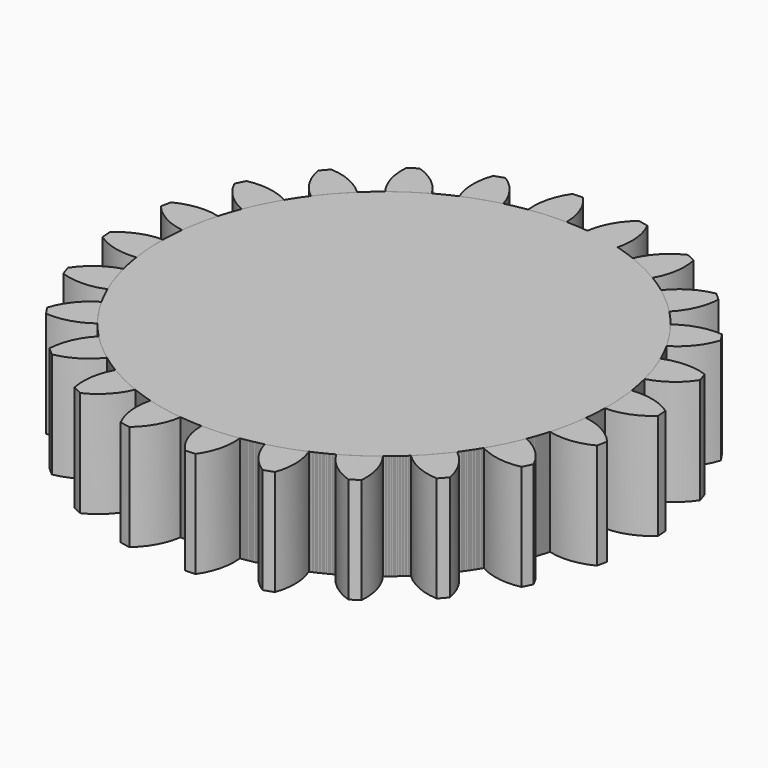
from build123d import *

# Parameters (mm, degrees)
F2_DEPTH = 1
F3_COUNT = 24
F3_ANGLE = 345


with BuildPart() as f2:
    # F1 (on Top) → F2 (new body)
    with BuildSketch(Plane.XY):
        with BuildLine():
            ThreePointArc((-0.3105516631, 2.0924649903), (-1.3816504371, -1.60184086), (2.1153846154, 0))
            ThreePointArc((2.1153846154, 0), (1.5080469337, 1.4834576222), (0.0347733631, 2.1150987883))
            ThreePointArc((0.0347733631, 2.1150987883), (-0.1383527734, 2.1108554145), (-0.3105516631, 2.0924649903))
        make_face()
        with BuildLine():
            ThreePointArc((-0.3105516631, 2.0924649903), (-0.1383527734, 2.1108554145), (0.0347733631, 2.1150987883))
            ThreePointArc((0.0347733631, 2.1150987883), (-0.0046162562, 2.3199411858), (-0.1142746835, 2.4973868937))
            ThreePointArc((-0.1142746835, 2.4973868937), (-0.1635078231, 2.4946473081), (-0.212677354, 2.4909372419))
            ThreePointArc((-0.212677354, 2.4909372419), (-0.2982363257, 2.3006963097), (-0.3105516631, 2.0924649903))
        make_face()
    extrude(amount=F2_DEPTH)


with BuildPart() as f3_1:
    # F3: instance of F2
    add(f2.part.rotate(Axis((0, 0, 1), (0, 0, 1)), 1 * F3_ANGLE / (F3_COUNT - 1)))


with BuildPart() as f3_2:
    # F3: instance of F2
    add(f2.part.rotate(Axis((0, 0, 1), (0, 0, 1)), 2 * F3_ANGLE / (F3_COUNT - 1)))


with BuildPart() as f3_3:
    # F3: instance of F2
    add(f2.part.rotate(Axis((0, 0, 1), (0, 0, 1)), 3 * F3_ANGLE / (F3_COUNT - 1)))


with BuildPart() as f3_4:
    # F3: instance of F2
    add(f2.part.rotate(Axis((0, 0, 1), (0, 0, 1)), 4 * F3_ANGLE / (F3_COUNT - 1)))


with BuildPart() as f3_5:
    # F3: instance of F2
    add(f2.part.rotate(Axis((0, 0, 1), (0, 0, 1)), 5 * F3_ANGLE / (F3_COUNT - 1)))


with BuildPart() as f3_6:
    # F3: instance of F2
    add(f2.part.rotate(Axis((0, 0, 1), (0, 0, 1)), 6 * F3_ANGLE / (F3_COUNT - 1)))


with BuildPart() as f3_7:
    # F3: instance of F2
    add(f2.part.rotate(Axis((0, 0, 1), (0, 0, 1)), 7 * F3_ANGLE / (F3_COUNT - 1)))


with BuildPart() as f3_8:
    # F3: instance of F2
    add(f2.part.rotate(Axis((0, 0, 1), (0, 0, 1)), 8 * F3_ANGLE / (F3_COUNT - 1)))


with BuildPart() as f3_9:
    # F3: instance of F2
    add(f2.part.rotate(Axis((0, 0, 1), (0, 0, 1)), 9 * F3_ANGLE / (F3_COUNT - 1)))


with BuildPart() as f3_10:
    # F3: instance of F2
    add(f2.part.rotate(Axis((0, 0, 1), (0, 0, 1)), 10 * F3_ANGLE / (F3_COUNT - 1)))


with BuildPart() as f3_11:
    # F3: instance of F2
    add(f2.part.rotate(Axis((0, 0, 1), (0, 0, 1)), 11 * F3_ANGLE / (F3_COUNT - 1)))


with BuildPart() as f3_12:
    # F3: instance of F2
    add(f2.part.rotate(Axis((0, 0, 1), (0, 0, 1)), 12 * F3_ANGLE / (F3_COUNT - 1)))


with BuildPart() as f3_13:
    # F3: instance of F2
    add(f2.part.rotate(Axis((0, 0, 1), (0, 0, 1)), 13 * F3_ANGLE / (F3_COUNT - 1)))


with BuildPart() as f3_14:
    # F3: instance of F2
    add(f2.part.rotate(Axis((0, 0, 1), (0, 0, 1)), 14 * F3_ANGLE / (F3_COUNT - 1)))


with BuildPart() as f3_15:
    # F3: instance of F2
    add(f2.part.rotate(Axis((0, 0, 1), (0, 0, 1)), 15 * F3_ANGLE / (F3_COUNT - 1)))


with BuildPart() as f3_16:
    # F3: instance of F2
    add(f2.part.rotate(Axis((0, 0, 1), (0, 0, 1)), 16 * F3_ANGLE / (F3_COUNT - 1)))


with BuildPart() as f3_17:
    # F3: instance of F2
    add(f2.part.rotate(Axis((0, 0, 1), (0, 0, 1)), 17 * F3_ANGLE / (F3_COUNT - 1)))


with BuildPart() as f3_18:
    # F3: instance of F2
    add(f2.part.rotate(Axis((0, 0, 1), (0, 0, 1)), 18 * F3_ANGLE / (F3_COUNT - 1)))


with BuildPart() as f3_19:
    # F3: instance of F2
    add(f2.part.rotate(Axis((0, 0, 1), (0, 0, 1)), 19 * F3_ANGLE / (F3_COUNT - 1)))


with BuildPart() as f3_20:
    # F3: instance of F2
    add(f2.part.rotate(Axis((0, 0, 1), (0, 0, 1)), 20 * F3_ANGLE / (F3_COUNT - 1)))


with BuildPart() as f3_21:
    # F3: instance of F2
    add(f2.part.rotate(Axis((0, 0, 1), (0, 0, 1)), 21 * F3_ANGLE / (F3_COUNT - 1)))


with BuildPart() as f3_22:
    # F3: instance of F2
    add(f2.part.rotate(Axis((0, 0, 1), (0, 0, 1)), 22 * F3_ANGLE / (F3_COUNT - 1)))


with BuildPart() as f3_23:
    # F3: instance of F2
    add(f2.part.rotate(Axis((0, 0, 1), (0, 0, 1)), 23 * F3_ANGLE / (F3_COUNT - 1)))


solid = Compound([f2.part, f3_1.part, f3_2.part, f3_3.part, f3_4.part, f3_5.part, f3_6.part, f3_7.part, f3_8.part, f3_9.part, f3_10.part, f3_11.part, f3_12.part, f3_13.part, f3_14.part, f3_15.part, f3_16.part, f3_17.part, f3_18.part, f3_19.part, f3_20.part, f3_21.part, f3_22.part, f3_23.part])
